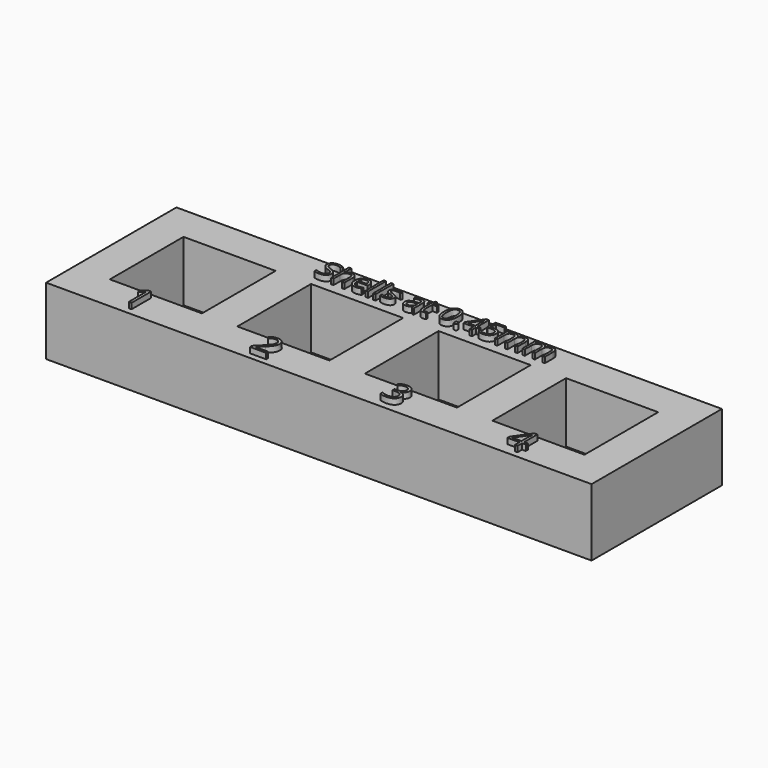
from build123d import *

# Parameters (mm, degrees)
F0_W           = 154
F0_H           = 46
F0_W_2         = 26
F0_H_2         = 26
F1_DEPTH       = 19
F2_DEPTH       = 17
F3_TEXT_SIZE   = 8.3107346048
F3_TEXT_SIZE_2 = 9.7222222222
F4_DEPTH       = 1.6


# Not quite as in the source:
# - Text() gives the source's letters only with a copy of the font that has no kerning and outlines rounded to 1/6400 em; it was checked with that copy


with BuildPart() as f1:
    # F0 (on Top) → F1 (new body)
    with BuildSketch(Plane.XY):
        with Locations((-77, 23)):
            Rectangle(F0_W, F0_H)
        with Locations((-131, 23)):
            Rectangle(F0_W_2, F0_H_2, mode=Mode.SUBTRACT)
        with Locations((-95, 23)):
            Rectangle(F0_W_2, F0_H_2, mode=Mode.SUBTRACT)
        with Locations((-59, 23)):
            Rectangle(F0_W_2, F0_H_2, mode=Mode.SUBTRACT)
        with Locations((-23, 23)):
            Rectangle(F0_W_2, F0_H_2, mode=Mode.SUBTRACT)
        with Locations((-131, 23)):
            Rectangle(F0_W_2, F0_H_2)
        with Locations((-95, 23)):
            Rectangle(F0_W_2, F0_H_2)
        with Locations((-59, 23)):
            Rectangle(F0_W_2, F0_H_2)
        with Locations((-23, 23)):
            Rectangle(F0_W_2, F0_H_2)
    extrude(amount=-F1_DEPTH)

    # F0 (on Top) → F2 (cut)
    with BuildSketch(Plane.XY):
        with Locations((-131, 23)):
            Rectangle(F0_W_2, F0_H_2)
        with Locations((-95, 23)):
            Rectangle(F0_W_2, F0_H_2)
        with Locations((-59, 23)):
            Rectangle(F0_W_2, F0_H_2)
        with Locations((-23, 23)):
            Rectangle(F0_W_2, F0_H_2)
    extrude(amount=-F2_DEPTH, mode=Mode.SUBTRACT)

    # F3 (on face) → F4 (join)
    with BuildSketch(Plane.XY):
        with Locations((-109.7222268581, 38.6502742767)):
            Text('Shells at 0.45mm', F3_TEXT_SIZE, font='Open Sans', text_align=(TextAlign.LEFT, TextAlign.BOTTOM))
        with Locations((-134.7415745258, 1.8344383985)):
            Text('1', F3_TEXT_SIZE_2, font='Open Sans', text_align=(TextAlign.LEFT, TextAlign.BOTTOM))
        with Locations((-98.2801765203, 1.7232491933)):
            Text('2', F3_TEXT_SIZE_2, font='Open Sans', text_align=(TextAlign.LEFT, TextAlign.BOTTOM))
        with Locations((-61.8676505983, 1.9743891731)):
            Text('3', F3_TEXT_SIZE_2, font='Open Sans', text_align=(TextAlign.LEFT, TextAlign.BOTTOM))
        with Locations((-26.5758093446, 1.694219403)):
            Text('4', F3_TEXT_SIZE_2, font='Open Sans', text_align=(TextAlign.LEFT, TextAlign.BOTTOM))
    extrude(amount=F4_DEPTH)


solid = f1.part
